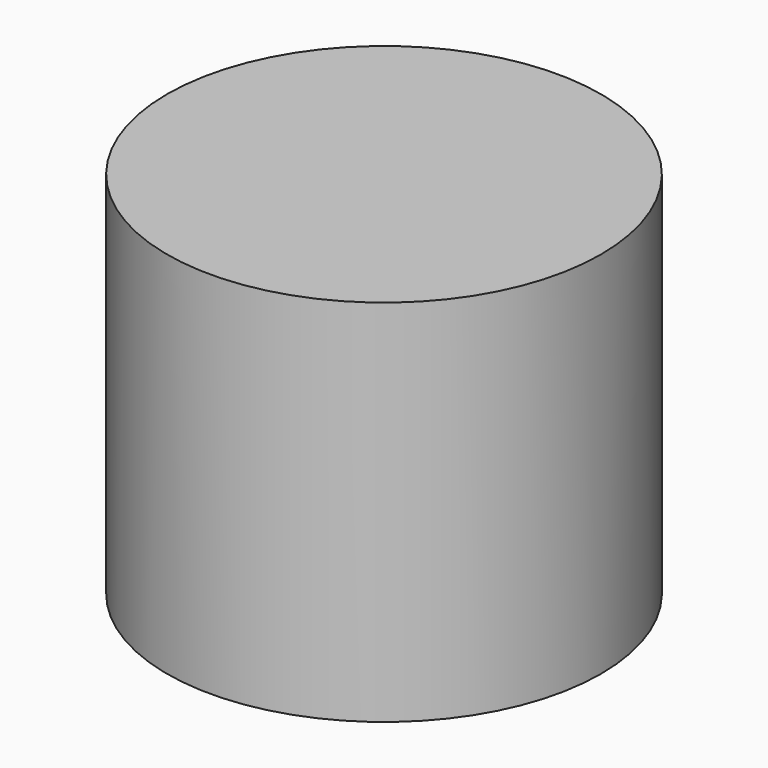
from build123d import *

# Parameters (mm, degrees)
F0_R     = 17.6314165874
F1_DEPTH = 30


# Not quite as in the source:
# - the program builds the solid bodies; features that only make, move or delete a surface that nothing else refers to are left out


with BuildPart() as f1:
    # F0 (on Top) → F1 (new body)
    with BuildSketch(Plane.XY):
        Circle(F0_R)
    extrude(amount=F1_DEPTH)


solid = f1.part
